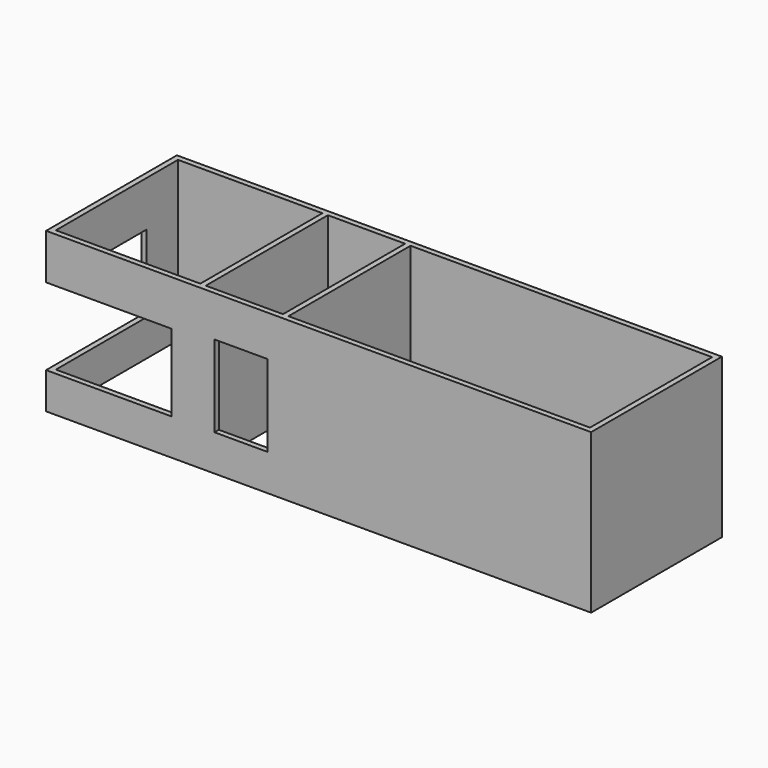
from build123d import *

# Parameters (mm, degrees)
F0_W      = 120
F0_H      = 36
F1_DEPTH  = 35
F2_W      = 7
F2_H      = 20
F3_DEPTH  = 1.2
F4_W      = 11.6417678248
F4_H      = 18
F5_DEPTH  = 1.201
F6_W      = 25
F6_H      = 17
F7_DEPTH  = 1.2
F8_W      = 1.2
F8_H      = 17
F9_DEPTH  = 3
F10_W     = 25
F10_H     = 17
F11_DEPTH = 1.2


with BuildPart() as f1:
    # F0 (on Top) → F1 (new body)
    with BuildSketch(Plane.XY):
        with Locations((-55.1781901717, -18)):
            Rectangle(F0_W, F0_H)
        Polygon((-113.9781901717, -34.8), (-113.9781901717, -1.2), (-107.9781901717, -1.2), (-89.9781901717, -1.2), (-82.1781901717, -1.2), (-80.9781901717, -1.2), (-63.9781901717, -1.2), (-62.7781901717, -1.2), (-49.0207746625, -1.2), (-45.235440135, -1.2), (3.6218098283, -1.2), (3.6218098283, -34.8), (-62.7781901717, -34.8), (-63.9781901717, -34.8), (-80.9781901717, -34.8), (-82.1781901717, -34.8), align=None, mode=Mode.SUBTRACT)
        Polygon((-82.1781901717, -26.7), (-82.1781901717, -34.8), (-80.9781901717, -34.8), (-80.9781901717, -26.6408454627), (-80.9781901717, -8.1258974969), (-80.9781901717, -1.2), (-82.1781901717, -1.2), (-82.1781901717, -8.7), align=None)
        Polygon((-63.9781901717, -26.6408454627), (-63.9781901717, -34.8), (-62.7781901717, -34.8), (-62.7781901717, -1.2), (-63.9781901717, -1.2), (-63.9781901717, -8.1258974969), align=None)
    extrude(amount=F1_DEPTH)

    # F2 (on face) → F3 (cut)
    with BuildSketch(Plane.YZ.offset(-80.9781901717)):
        with Locations((-5.5, 10)):
            Rectangle(F2_W, F2_H)
    extrude(amount=-F3_DEPTH, mode=Mode.SUBTRACT)

    # F4 (on face) → F5 (cut, through all)
    with BuildSketch(Plane(origin=(0, -34.8, 0), x_dir=(-1, 0, 0), z_dir=(0, 1, 0))):
        with Locations((72.271104902, 17)):
            Rectangle(F4_W, F4_H)
    extrude(amount=-F5_DEPTH, mode=Mode.SUBTRACT)

    # F6 (on face) → F7 (cut)
    with BuildSketch(Plane(origin=(0, -34.8, 0), x_dir=(-1, 0, 0), z_dir=(0, 1, 0))):
        with Locations((100.0405803323, 16.5)):
            Rectangle(F6_W, F6_H)
    extrude(amount=-F7_DEPTH, mode=Mode.SUBTRACT)

    # F8 (on face) → F9 (cut)
    with BuildSketch(Plane.YZ.offset(-112.5405803323)):
        with Locations((-35.4, 16.5)):
            Rectangle(F8_W, F8_H)
    extrude(amount=-F9_DEPTH, mode=Mode.SUBTRACT)

    # F10 (on face) → F11 (cut)
    with BuildSketch(Plane(origin=(-115.1781901717, 0, 0), x_dir=(0, -1, 0), z_dir=(-1, 0, 0))):
        with Locations((22.3, 16.5)):
            Rectangle(F10_W, F10_H)
    extrude(amount=-F11_DEPTH, mode=Mode.SUBTRACT)


solid = f1.part
